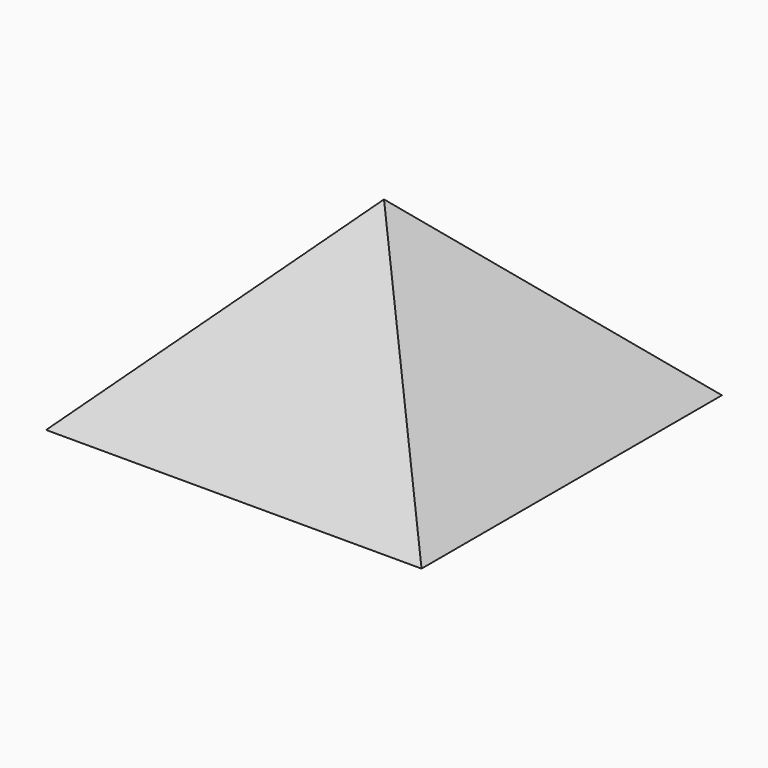
from build123d import *

# Parameters (mm, degrees)
F0_W     = 10
F0_H     = 10
F1_DEPTH = 5
F2_SIZE  = 4.99999


# Not quite as in the source:
# - a fillet or chamfer is up to 0.001 mm smaller than in the source, because OpenCascade refuses the exact size


with BuildPart() as f1:
    # F0 (on Top) → F1 (new body)
    with BuildSketch(Plane.XY):
        Rectangle(F0_W, F0_H)
    extrude(amount=F1_DEPTH)

    # F2 (size 5 in the source; OpenCascade refuses exactly that, so slightly less here)
    f2_edges = [f1.edges().sort_by_distance(p)[0] for p in [
        (-5, 0, 5),
        (0, -5, 5),
        (5, 0, 5),
        (0, 5, 5),
    ]]
    chamfer(f2_edges, length=F2_SIZE)


solid = f1.part
